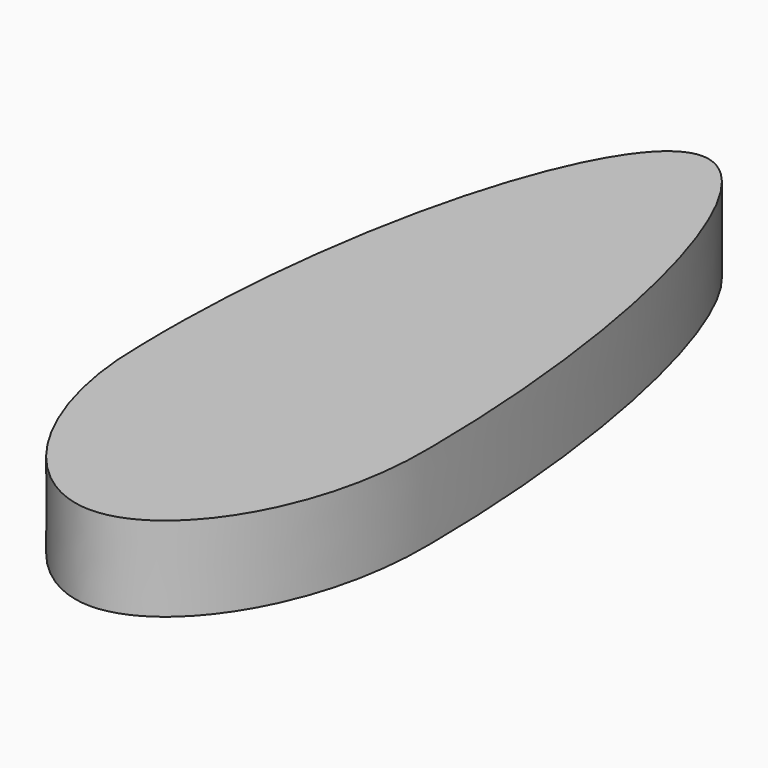
from build123d import *

# Parameters (mm, degrees)
F4_DEPTH = 410


# Not quite as in the source:
# - the program builds the solid bodies; features that only make, move or delete a surface that nothing else refers to are left out


with BuildPart() as f4:
    # F2 (on plane+point) → F4 (new body)
    with BuildSketch(Plane.XY.offset(410)):
        with BuildLine():
            Line((689.1178958249, 0), (0, 0))
            Line((0, 0), (0, -1162))
            add(Edge.make_bspline(
                [(0, -1162), (344.5589479125, -1165.0347502999), (689.1178958249, -651.2407064438), (689.1178958249, 0)],
                knots=[0.5, 0.5, 0.5, 0.5, 1, 1, 1, 1], degree=3))
        make_face()
        with BuildLine():
            Line((0, 2545), (0, 0))
            Line((0, 0), (689.1178958249, 0))
            add(Edge.make_bspline(
                [(689.1178958249, 0), (689.1178958249, 1292.9308553383), (352.9144642907, 2543.0320965212), (0, 2545)],
                knots=[0, 0, 0, 0, 0.5, 0.5, 0.5, 0.5], degree=3))
        make_face()
        with BuildLine():
            Line((0, -1162), (0, 0))
            Line((0, 0), (-689.1178958249, 0))
            add(Edge.make_bspline(
                [(-689.1178958249, 0), (-689.1178958249, -639.1017052442), (-344.5589479125, -1158.9652497001), (0, -1162)],
                knots=[0, 0, 0, 0, 0.5, 0.5, 0.5, 0.5], degree=3))
        make_face()
        with BuildLine():
            Line((-689.1178958249, 0), (0, 0))
            Line((0, 0), (0, 2545))
            add(Edge.make_bspline(
                [(0, 2545), (-352.9144642907, 2546.9679034788), (-722.539961338, 1300.8024692535), (-689.1178958249, 0)],
                knots=[0.5, 0.5, 0.5, 0.5, 1, 1, 1, 1], degree=3))
        make_face()
    extrude(amount=-F4_DEPTH)


solid = f4.part
